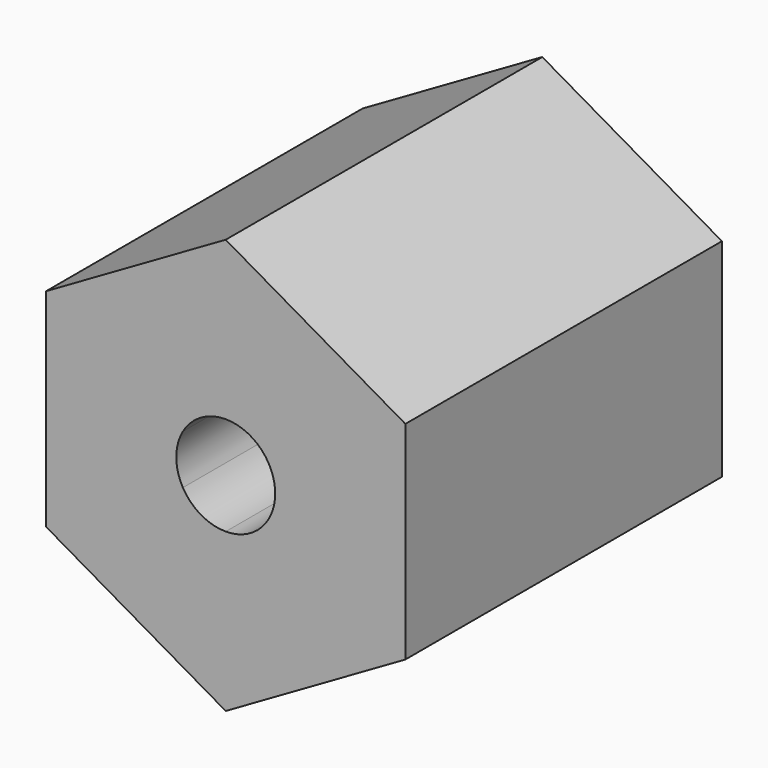
from build123d import *

# Parameters (mm, degrees)
F1_DEPTH = 12.7


# Not quite as in the source:
# - a feature names something its author has since deleted; it is built from what else it names


with BuildPart() as f1:
    # F0 (on Front) → F1 (new body)
    with BuildSketch(Plane.XZ):
        Polygon((5.7657995114, 3.3288859), (0, 6.6577718), (-5.7657995114, 3.3288859), (-5.7657995114, -3.3288859), (0, -6.6577718), (5.7657995114, -3.3288859), align=None)
        with BuildLine():
            ThreePointArc((-1.3748153285, 0.79375), (-0.79375, 1.3748153285), (0, 1.5875))
            ThreePointArc((0, 1.5875), (0.79375, 1.3748153285), (1.3748153285, 0.79375))
            ThreePointArc((1.3748153285, 0.79375), (1.5334072492, 0.4108752341), (1.5875, 0))
            ThreePointArc((1.5875, 0), (1.5334072492, -0.4108752341), (1.3748153285, -0.79375))
            ThreePointArc((1.3748153285, -0.79375), (0.79375, -1.3748153285), (0, -1.5875))
            ThreePointArc((0, -1.5875), (-0.79375, -1.3748153285), (-1.3748153285, -0.79375))
            ThreePointArc((-1.3748153285, -0.79375), (-1.5875, 0), (-1.3748153285, 0.79375))
        make_face(mode=Mode.SUBTRACT)
    extrude(amount=F1_DEPTH)


solid = f1.part
